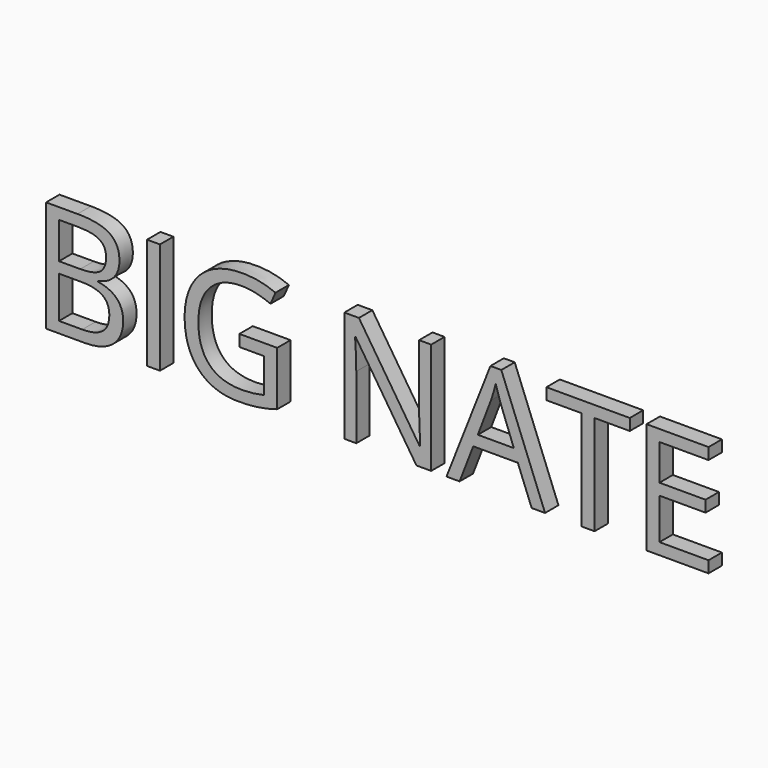
from build123d import *

# Parameters (mm, degrees)
F0_TEXT_SIZE = 59.0594407792
F1_DEPTH     = 6.35


# Not quite as in the source:
# - Text() gives the source's letters only with a copy of the font that has no kerning and outlines rounded to 1/6400 em; it was checked with that copy


with BuildPart() as f1:
    # F0 (on Front) → F1 (new body)
    with BuildSketch(Plane.XZ):
        with Locations((-134.9923759699, -25.9099602699)):
            Text('BIG NATE', F0_TEXT_SIZE, font='Open Sans', text_align=(TextAlign.LEFT, TextAlign.BOTTOM))
    extrude(amount=F1_DEPTH)


solid = f1.part
